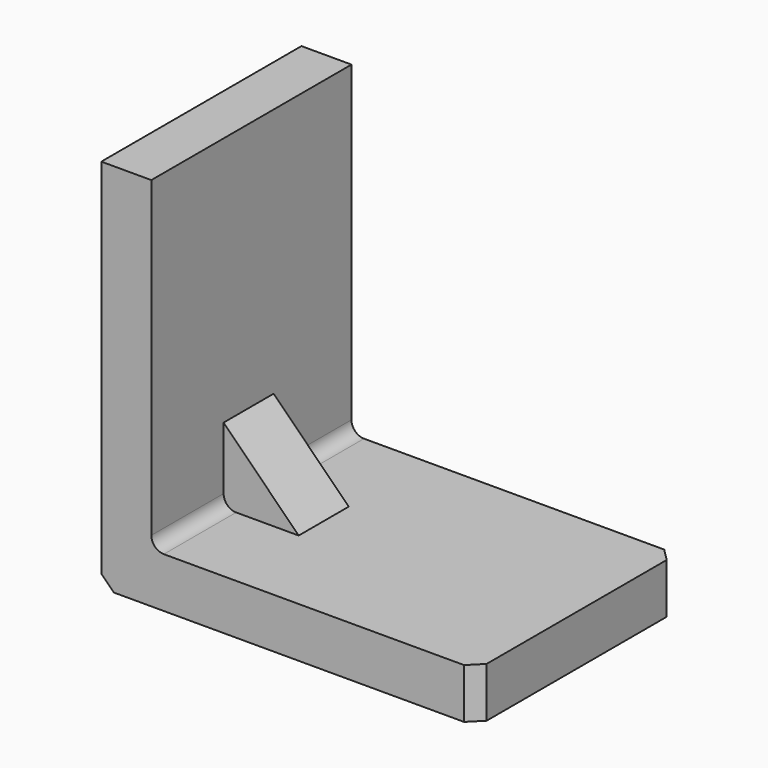
from build123d import *

# Parameters (mm, degrees)
F0_W      = 300
F0_H      = 200
F1_DEPTH  = 300
F2_W      = 260
F2_H      = 200
F3_DEPTH  = 260
F4_R      = 10
F5_W      = 60
F5_H      = 50
F6_DEPTH  = 260
F7_SIZE   = 10
F8_W      = 60
F8_H      = 50
F9_DEPTH  = 200
F11_DEPTH = 50


# Not quite as in the source:
# - a feature names something its author has since deleted; it is built from what else it names


with BuildPart() as f1:
    # F0 (on Top) → F1 (new body)
    with BuildSketch(Plane.XY):
        with Locations((-1.4433003962, 18.309512734)):
            Rectangle(F0_W, F0_H)
    extrude(amount=F1_DEPTH)

    # F2 (on face) → F3 (cut)
    with BuildSketch(Plane.XY.offset(300)):
        with Locations((18.5566996038, 18.309512734)):
            Rectangle(F2_W, F2_H)
    extrude(amount=-F3_DEPTH, mode=Mode.SUBTRACT)

    # F4
    f4_edges = [f1.edges().sort_by_distance(p)[0] for p in [
        (-111.4433, 18.309513, 40),
    ]]
    fillet(f4_edges, radius=F4_R)

    # F5 (on face) → F6 (join)
    with BuildSketch(Plane.XY.offset(300)):
        with Locations((-81.4433003962, 15.5513301492)):
            Rectangle(F5_W, F5_H)
    extrude(amount=-F6_DEPTH)

    # F7
    f7_edges = [f1.edges().sort_by_distance(p)[0] for p in [
        (-151.4433, 18.309513, 0),
        (148.5567, -81.690487, 20),
        (148.5567, 118.309513, 20),
    ]]
    chamfer(f7_edges, length=F7_SIZE)

    # F8 (on face) → F9 (cut)
    with BuildSketch(Plane.XY.offset(300)):
        with Locations((-81.4433003962, 15.5513301492)):
            Rectangle(F8_W, F8_H)
    extrude(amount=-F9_DEPTH, mode=Mode.SUBTRACT)

    # F10 (on face) → F11 (cut)
    with BuildSketch(Plane.XZ.offset(9.4486698508)):
        Polygon((-51.4433003962, 100), (-111.4433003962, 100), (-51.4433003962, 40), align=None)
    extrude(amount=-F11_DEPTH, mode=Mode.SUBTRACT)


solid = f1.part
